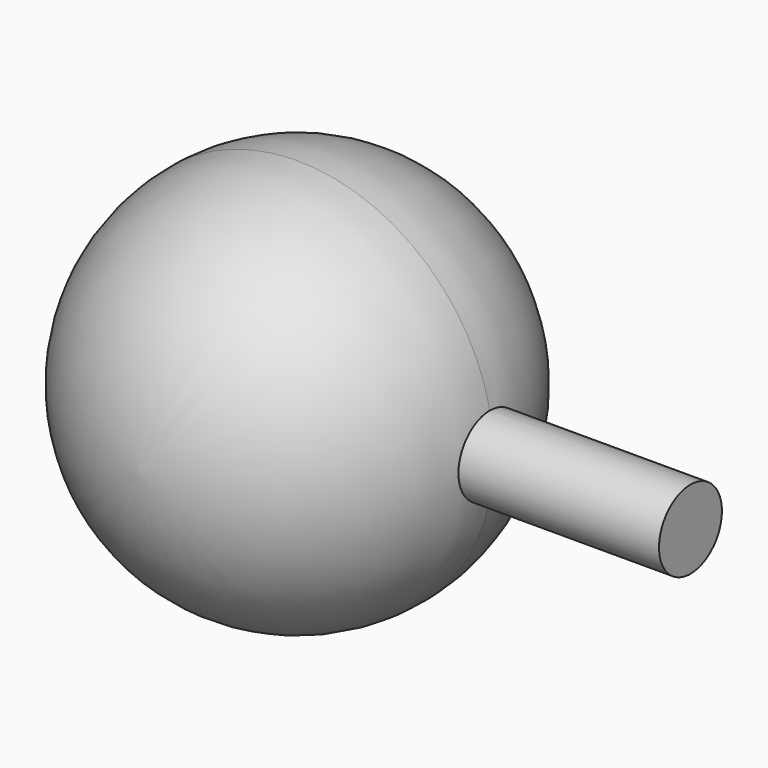
from build123d import *

# Parameters (mm, degrees)
F0_R     = 12.5
F1_DEPTH = 12.5
F2_R     = 12.49999
F3_R     = 2.5
F4_DEPTH = 25


# Not quite as in the source:
# - a fillet or chamfer is up to 0.001 mm smaller than in the source, because OpenCascade refuses the exact size


with BuildPart() as f1:
    # F0 (on Front) → F1 (new body, symmetric)
    with BuildSketch(Plane.XZ):
        Circle(F0_R)
    extrude(amount=F1_DEPTH, both=True)

    # F2 (radius 12.5 in the source; OpenCascade refuses exactly that, so slightly less here)
    f2_edges = [f1.edges().sort_by_distance(p)[0] for p in [
        (-12.5, -12.5, 0),
        (-12.5, 12.5, 0),
    ]]
    fillet(f2_edges, radius=F2_R)

    # F3 (on Right) → F4 (join)
    with BuildSketch(Plane.YZ):
        Circle(F3_R)
    extrude(amount=F4_DEPTH)


solid = f1.part
